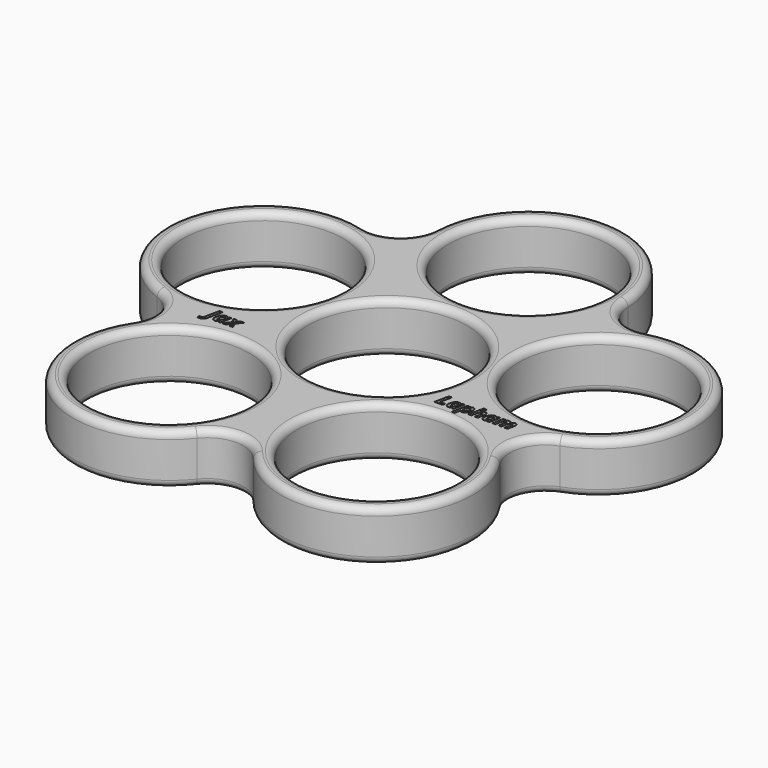
from build123d import *

# Parameters (mm, degrees)
F0_R         = 11.125
F1_DEPTH     = 7
F2_R         = 1
F3_TEXT_SIZE = 2.8943560058
F4_DEPTH     = 0.5
F5_TEXT_SIZE = 2.7777777778
F6_DEPTH     = 0.5


# Not quite as in the source:
# - Text() gives the source's letters only with a copy of the font that has no kerning and outlines rounded to 1/6400 em; it was checked with that copy


with BuildPart() as f1:
    # F0 (on Top) → F1 (new body)
    with BuildSketch(Plane.XY):
        with BuildLine():
            ThreePointArc((19.7488320667, 20.5197915807), (15.4692706439, 21.2916244371), (13.4127567682, 25.1232197458))
            ThreePointArc((13.4127567682, 25.1232197458), (0, 37.975), (-13.4127567682, 25.1232197458))
            ThreePointArc((-13.4127567682, 25.1232197458), (-15.4692706439, 21.2916244371), (-19.7488320667, 20.5197915807))
            ThreePointArc((-19.7488320667, 20.5197915807), (-36.1163712063, 11.7349203614), (-28.0383716323, -4.992787871))
            ThreePointArc((-28.0383716323, -4.992787871), (-25.029805683, -8.1326768593), (-25.6182062236, -12.4412911068))
            ThreePointArc((-25.6182062236, -12.4412911068), (-22.3211449558, -30.7224203614), (-3.9159098898, -28.2089323487))
            ThreePointArc((-3.9159098898, -28.2089323487), (0, -26.3178951557), (3.9159098898, -28.2089323487))
            ThreePointArc((3.9159098898, -28.2089323487), (22.3211449558, -30.7224203614), (25.6182062236, -12.4412911068))
            ThreePointArc((25.6182062236, -12.4412911068), (25.029805683, -8.1326768593), (28.0383716323, -4.992787871))
            ThreePointArc((28.0383716323, -4.992787871), (36.1163712063, 11.7349203614), (19.7488320667, 20.5197915807))
        make_face()
        with Locations((-14.4301279438, -19.8613672119)):
            Circle(F0_R, mode=Mode.SUBTRACT)
        with Locations((14.4301279438, -19.8613672119)):
            Circle(F0_R, mode=Mode.SUBTRACT)
        Circle(F0_R, mode=Mode.SUBTRACT)
        with Locations((-23.348437475, 7.5863672119)):
            Circle(F0_R, mode=Mode.SUBTRACT)
        with Locations((23.348437475, 7.5863672119)):
            Circle(F0_R, mode=Mode.SUBTRACT)
        with Locations((0, 24.55)):
            Circle(F0_R, mode=Mode.SUBTRACT)
    extrude(amount=F1_DEPTH)

    # F2
    f2_edges = [f1.edges().sort_by_distance(p)[0] for p in [
        (-36.116371, 11.73492, 7),
        (-22.321145, -30.72242, 0),
        (-25.555128, -19.861367, 7),
        (-34.473437, 7.586367, 7),
        (-11.125, 24.55, 0),
        (-11.125, 24.55, 7),
        (-34.473437, 7.586367, 0),
        (-25.555128, -19.861367, 0),
        (-11.125, 0, 0),
        (-11.125, 0, 7),
        (12.223437, 7.586367, 0),
        (12.223437, 7.586367, 7),
        (3.305128, -19.861367, 0),
        (3.305128, -19.861367, 7),
    ]]
    fillet(f2_edges, radius=F2_R)

    # F3 (on face) → F4 (cut)
    with BuildSketch(Plane.XY.offset(7)):
        with Locations((-20.0548249884, -6.8530899032)):
            Text('Jax', F3_TEXT_SIZE, font='Open Sans', font_style=FontStyle.BOLDITALIC, text_align=(TextAlign.LEFT, TextAlign.BOTTOM))
    extrude(amount=-F4_DEPTH, mode=Mode.SUBTRACT)

    # F5 (on face) → F6 (cut)
    with BuildSketch(Plane.XY.offset(7)):
        with Locations((12.0105272222, -6.8889808413)):
            Text('Lapham', F5_TEXT_SIZE, font='Open Sans', font_style=FontStyle.BOLDITALIC, text_align=(TextAlign.LEFT, TextAlign.BOTTOM))
    extrude(amount=-F6_DEPTH, mode=Mode.SUBTRACT)


solid = f1.part
